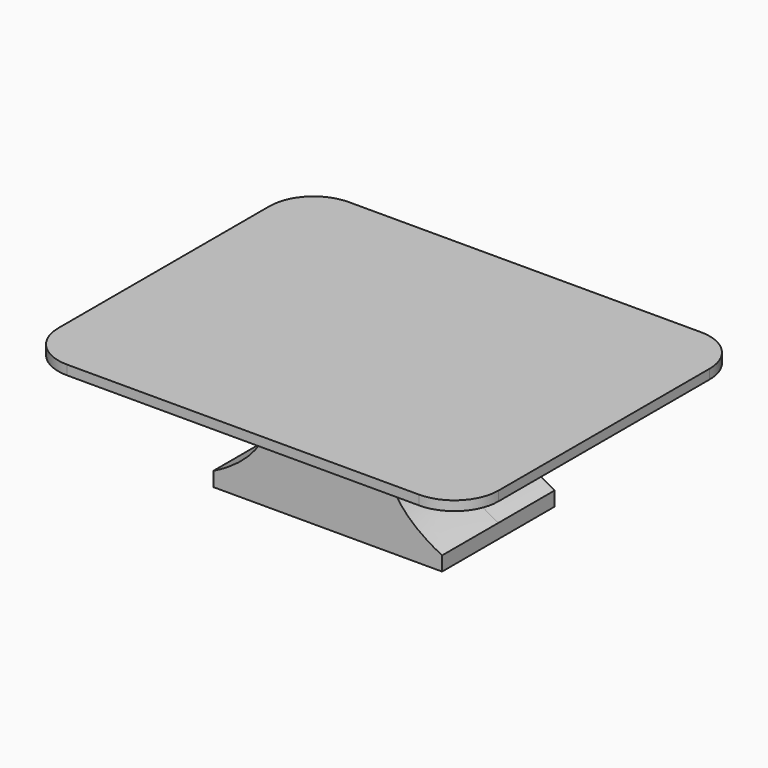
from build123d import *

# Parameters (mm, degrees)
F1_DEPTH     = 20
F2_DEPTH     = 13
F0_W         = 13
F0_H         = 1.6210871795
F3_T4_DEPTH  = 22
F3_T9_DEPTH  = 26
F3_T14_DEPTH = 26
F3_T19_DEPTH = 22
F3_T25_DEPTH = 38.8584149398
F3_T30_DEPTH = 34.8584149398
F3_T38_DEPTH = 34.8584149398
F3_T43_DEPTH = 38.8584149398
F3_T51_DEPTH = 38.8584149398
F3_T56_DEPTH = 34.8584149398
F3_T64_DEPTH = 38.8584149398
F3_T69_DEPTH = 34.8584149398
F4_R         = 5
F5_R         = 5
F7_DEPTH     = 8


# Not quite as in the source:
# - a fillet or chamfer that OpenCascade refuses, or shapes differently, is made with other operations: its cross-section is extruded or revolved along the edge and cut away or added


with BuildPart() as f1:
    # F0 (on Front) → F1 (new body, symmetric)
    with BuildSketch(Plane.XZ):
        Polygon((0, 13.7715177082), (0, 14.85), (-25, 14.85), (-25, 13.7715177082), (-11, 13.7715177082), align=None)
        Polygon((25, 14.85), (0, 14.85), (0, 13.7715177082), (11, 13.7715177082), (25, 13.7715177082), align=None)
    extrude(amount=F1_DEPTH, both=True)

    # F0 (on Front) → F2 (join, symmetric)
    with BuildSketch(Plane.XZ):
        Polygon((0, 12.6210871795), (0, 13.7715177082), (-11, 13.7715177082), (-11, 12.6210871795), (-5.5, 12.6210871795), align=None)
        Polygon((11, 13.7715177082), (0, 13.7715177082), (0, 12.6210871795), (5.5, 12.6210871795), (11, 12.6210871795), align=None)
    extrude(amount=F2_DEPTH, both=True)

    # F3: chamfer of 5 on 4 edges, made by hand


with BuildPart() as f2:
    # F0 (on Front) → F2, piece 2 (new body, symmetric)
    with BuildSketch(Plane.XZ):
        with Locations((-6.5, 0.8105435898)):
            Rectangle(F0_W, F0_H)
        with Locations((6.5, 0.8105435898)):
            Rectangle(F0_W, F0_H)
    extrude(amount=F2_DEPTH, both=True)

    # F4
    f4_edges = [f2.edges().sort_by_distance(p)[0] for p in [
        (-13, 13, 0.810544),
        (-13, -13, 0.810544),
        (13, -13, 0.810544),
        (13, 13, 0.810544),
    ]]
    fillet(f4_edges, radius=F4_R)


with BuildPart() as f3_tool2:
    # F3_s3 → F3_t4 (new body)
    with BuildSketch(Plane.YZ.offset(-11)):
        with BuildLine():
            Line((13.1414213562, 17.7625085358), (7.8585786438, 12.4796658233))
            Line((7.8585786438, 12.4796658233), (7.8585786438, 12.3796658233))
            ThreePointArc((7.8585786438, 12.3796658233), (10.4292893219, 12.5210871795), (13, 12.5210871795))
            Line((13, 12.5210871795), (13.1, 12.6210871795))
            ThreePointArc((13.1, 12.6210871795), (13.1, 15.1917978577), (13.2414213562, 17.7625085358))
            Line((13.2414213562, 17.7625085358), (13.1414213562, 17.7625085358))
        make_face()
    extrude(amount=F3_T4_DEPTH)

    split(bisect_by=Plane.XY.offset(13.7715177082), keep=Keep.BOTTOM)


with BuildPart() as f1_1:
    add(f1.part)

    # F3_t1: cut F3_tool2
    add(f3_tool2.part, mode=Mode.SUBTRACT)


with BuildPart() as f3_tool7:
    # F3_s8 → F3_t9 (new body)
    with BuildSketch(Plane.XZ.offset(-13)):
        with BuildLine():
            Line((-11.1414213562, 17.7625085358), (-5.8585786438, 12.4796658233))
            Line((-5.8585786438, 12.4796658233), (-5.8585786438, 12.3796658233))
            ThreePointArc((-5.8585786438, 12.3796658233), (-8.4292893219, 12.5210871795), (-11, 12.5210871795))
            Line((-11, 12.5210871795), (-11.1, 12.6210871795))
            ThreePointArc((-11.1, 12.6210871795), (-11.1, 15.1917978577), (-11.2414213562, 17.7625085358))
            Line((-11.2414213562, 17.7625085358), (-11.1414213562, 17.7625085358))
        make_face()
    extrude(amount=F3_T9_DEPTH)

    split(bisect_by=Plane.XY.offset(13.7715177082), keep=Keep.BOTTOM)


with BuildPart() as f1_2:
    add(f1_1.part)

    # F3_t6: cut F3_tool7
    add(f3_tool7.part, mode=Mode.SUBTRACT)


with BuildPart() as f3_tool12:
    # F3_s13 → F3_t14 (new body)
    with BuildSketch(Plane.XZ.offset(-13)):
        with BuildLine():
            Line((11.1414213562, 17.7625085358), (5.8585786438, 12.4796658233))
            Line((5.8585786438, 12.4796658233), (5.8585786438, 12.3796658233))
            ThreePointArc((5.8585786438, 12.3796658233), (8.4292893219, 12.5210871795), (11, 12.5210871795))
            Line((11, 12.5210871795), (11.1, 12.6210871795))
            ThreePointArc((11.1, 12.6210871795), (11.1, 15.1917978577), (11.2414213562, 17.7625085358))
            Line((11.2414213562, 17.7625085358), (11.1414213562, 17.7625085358))
        make_face()
    extrude(amount=F3_T14_DEPTH)

    split(bisect_by=Plane.XY.offset(13.7715177082), keep=Keep.BOTTOM)


with BuildPart() as f1_3:
    add(f1_2.part)

    # F3_t11: cut F3_tool12
    add(f3_tool12.part, mode=Mode.SUBTRACT)


with BuildPart() as f3_tool17:
    # F3_s18 → F3_t19 (new body)
    with BuildSketch(Plane.YZ.offset(-11)):
        with BuildLine():
            Line((-13.1414213562, 17.7625085358), (-7.8585786438, 12.4796658233))
            Line((-7.8585786438, 12.4796658233), (-7.8585786438, 12.3796658233))
            ThreePointArc((-7.8585786438, 12.3796658233), (-10.4292893219, 12.5210871795), (-13, 12.5210871795))
            Line((-13, 12.5210871795), (-13.1, 12.6210871795))
            ThreePointArc((-13.1, 12.6210871795), (-13.1, 15.1917978577), (-13.2414213562, 17.7625085358))
            Line((-13.2414213562, 17.7625085358), (-13.1414213562, 17.7625085358))
        make_face()
    extrude(amount=F3_T19_DEPTH)

    split(bisect_by=Plane.XY.offset(13.7715177082), keep=Keep.BOTTOM)


with BuildPart() as f1_4:
    add(f1_3.part)

    # F3_t16: cut F3_tool17
    add(f3_tool17.part, mode=Mode.SUBTRACT)


with BuildPart() as f3_tool23:
    # F3_s24 → F3_t25 (new body)
    with BuildSketch(Plane.XZ.offset(-25.8584149398)):
        with BuildLine():
            Line((-11.1414213562, 17.7625085358), (-5.8585786438, 12.4796658233))
            Line((-5.8585786438, 12.4796658233), (-5.8585786438, 12.3796658233))
            ThreePointArc((-5.8585786438, 12.3796658233), (-8.4292893219, 12.5210871795), (-11, 12.5210871795))
            Line((-11, 12.5210871795), (-11.1, 12.6210871795))
            ThreePointArc((-11.1, 12.6210871795), (-11.1, 15.1917978577), (-11.2414213562, 17.7625085358))
            Line((-11.2414213562, 17.7625085358), (-11.1414213562, 17.7625085358))
        make_face()
    extrude(amount=F3_T25_DEPTH)

    split(bisect_by=Plane.XY.offset(13.7715177082), keep=Keep.BOTTOM)

    split(bisect_by=Plane.XZ.offset(-13), keep=Keep.BOTTOM)


with BuildPart() as f3_tool28:
    # F3_s29 → F3_t30 (new body)
    with BuildSketch(Plane.YZ.offset(-23.8584149398)):
        with BuildLine():
            Line((13.1414213562, 17.7625085358), (7.8585786438, 12.4796658233))
            Line((7.8585786438, 12.4796658233), (7.8585786438, 12.3796658233))
            ThreePointArc((7.8585786438, 12.3796658233), (10.4292893219, 12.5210871795), (13, 12.5210871795))
            Line((13, 12.5210871795), (13.1, 12.6210871795))
            ThreePointArc((13.1, 12.6210871795), (13.1, 15.1917978577), (13.2414213562, 17.7625085358))
            Line((13.2414213562, 17.7625085358), (13.1414213562, 17.7625085358))
        make_face()
    extrude(amount=F3_T30_DEPTH)

    split(bisect_by=Plane.XY.offset(13.7715177082), keep=Keep.BOTTOM)

    split(bisect_by=Plane.YZ.offset(-11), keep=Keep.BOTTOM)


with BuildPart() as f3_tool23_1:
    add(f3_tool23.part)

    # F3_t33: intersect F3_tool28
    add(f3_tool28.part, mode=Mode.INTERSECT)


with BuildPart() as f1_5:
    add(f1_4.part)

    # F3_t21: cut F3_tool23
    add(f3_tool23_1.part, mode=Mode.SUBTRACT)


with BuildPart() as f3_tool36:
    # F3_s37 → F3_t38 (new body)
    with BuildSketch(Plane.YZ.offset(-11)):
        with BuildLine():
            Line((13.1414213562, 17.7625085358), (7.8585786438, 12.4796658233))
            Line((7.8585786438, 12.4796658233), (7.8585786438, 12.3796658233))
            ThreePointArc((7.8585786438, 12.3796658233), (10.4292893219, 12.5210871795), (13, 12.5210871795))
            Line((13, 12.5210871795), (13.1, 12.6210871795))
            ThreePointArc((13.1, 12.6210871795), (13.1, 15.1917978577), (13.2414213562, 17.7625085358))
            Line((13.2414213562, 17.7625085358), (13.1414213562, 17.7625085358))
        make_face()
    extrude(amount=F3_T38_DEPTH)

    split(bisect_by=Plane.XY.offset(13.7715177082), keep=Keep.BOTTOM)

    split(bisect_by=Plane.YZ.offset(11), keep=Keep.TOP)


with BuildPart() as f3_tool41:
    # F3_s42 → F3_t43 (new body)
    with BuildSketch(Plane.XZ.offset(-25.8584149398)):
        with BuildLine():
            Line((11.1414213562, 17.7625085358), (5.8585786438, 12.4796658233))
            Line((5.8585786438, 12.4796658233), (5.8585786438, 12.3796658233))
            ThreePointArc((5.8585786438, 12.3796658233), (8.4292893219, 12.5210871795), (11, 12.5210871795))
            Line((11, 12.5210871795), (11.1, 12.6210871795))
            ThreePointArc((11.1, 12.6210871795), (11.1, 15.1917978577), (11.2414213562, 17.7625085358))
            Line((11.2414213562, 17.7625085358), (11.1414213562, 17.7625085358))
        make_face()
    extrude(amount=F3_T43_DEPTH)

    split(bisect_by=Plane.XY.offset(13.7715177082), keep=Keep.BOTTOM)

    split(bisect_by=Plane.XZ.offset(-13), keep=Keep.BOTTOM)


with BuildPart() as f3_tool36_1:
    add(f3_tool36.part)

    # F3_t46: intersect F3_tool41
    add(f3_tool41.part, mode=Mode.INTERSECT)


with BuildPart() as f1_6:
    add(f1_5.part)

    # F3_t34: cut F3_tool36
    add(f3_tool36_1.part, mode=Mode.SUBTRACT)


with BuildPart() as f3_tool49:
    # F3_s50 → F3_t51 (new body)
    with BuildSketch(Plane.XZ.offset(-13)):
        with BuildLine():
            Line((-11.1414213562, 17.7625085358), (-5.8585786438, 12.4796658233))
            Line((-5.8585786438, 12.4796658233), (-5.8585786438, 12.3796658233))
            ThreePointArc((-5.8585786438, 12.3796658233), (-8.4292893219, 12.5210871795), (-11, 12.5210871795))
            Line((-11, 12.5210871795), (-11.1, 12.6210871795))
            ThreePointArc((-11.1, 12.6210871795), (-11.1, 15.1917978577), (-11.2414213562, 17.7625085358))
            Line((-11.2414213562, 17.7625085358), (-11.1414213562, 17.7625085358))
        make_face()
    extrude(amount=F3_T51_DEPTH)

    split(bisect_by=Plane.XY.offset(13.7715177082), keep=Keep.BOTTOM)

    split(bisect_by=Plane.XZ.offset(13), keep=Keep.TOP)


with BuildPart() as f3_tool54:
    # F3_s55 → F3_t56 (new body)
    with BuildSketch(Plane.YZ.offset(-23.8584149398)):
        with BuildLine():
            Line((-13.1414213562, 17.7625085358), (-7.8585786438, 12.4796658233))
            Line((-7.8585786438, 12.4796658233), (-7.8585786438, 12.3796658233))
            ThreePointArc((-7.8585786438, 12.3796658233), (-10.4292893219, 12.5210871795), (-13, 12.5210871795))
            Line((-13, 12.5210871795), (-13.1, 12.6210871795))
            ThreePointArc((-13.1, 12.6210871795), (-13.1, 15.1917978577), (-13.2414213562, 17.7625085358))
            Line((-13.2414213562, 17.7625085358), (-13.1414213562, 17.7625085358))
        make_face()
    extrude(amount=F3_T56_DEPTH)

    split(bisect_by=Plane.XY.offset(13.7715177082), keep=Keep.BOTTOM)

    split(bisect_by=Plane.YZ.offset(-11), keep=Keep.BOTTOM)


with BuildPart() as f3_tool49_1:
    add(f3_tool49.part)

    # F3_t59: intersect F3_tool54
    add(f3_tool54.part, mode=Mode.INTERSECT)


with BuildPart() as f1_7:
    add(f1_6.part)

    # F3_t47: cut F3_tool49
    add(f3_tool49_1.part, mode=Mode.SUBTRACT)


with BuildPart() as f3_tool62:
    # F3_s63 → F3_t64 (new body)
    with BuildSketch(Plane.XZ.offset(-13)):
        with BuildLine():
            Line((11.1414213562, 17.7625085358), (5.8585786438, 12.4796658233))
            Line((5.8585786438, 12.4796658233), (5.8585786438, 12.3796658233))
            ThreePointArc((5.8585786438, 12.3796658233), (8.4292893219, 12.5210871795), (11, 12.5210871795))
            Line((11, 12.5210871795), (11.1, 12.6210871795))
            ThreePointArc((11.1, 12.6210871795), (11.1, 15.1917978577), (11.2414213562, 17.7625085358))
            Line((11.2414213562, 17.7625085358), (11.1414213562, 17.7625085358))
        make_face()
    extrude(amount=F3_T64_DEPTH)

    split(bisect_by=Plane.XY.offset(13.7715177082), keep=Keep.BOTTOM)

    split(bisect_by=Plane.XZ.offset(13), keep=Keep.TOP)


with BuildPart() as f3_tool67:
    # F3_s68 → F3_t69 (new body)
    with BuildSketch(Plane.YZ.offset(-11)):
        with BuildLine():
            Line((-13.1414213562, 17.7625085358), (-7.8585786438, 12.4796658233))
            Line((-7.8585786438, 12.4796658233), (-7.8585786438, 12.3796658233))
            ThreePointArc((-7.8585786438, 12.3796658233), (-10.4292893219, 12.5210871795), (-13, 12.5210871795))
            Line((-13, 12.5210871795), (-13.1, 12.6210871795))
            ThreePointArc((-13.1, 12.6210871795), (-13.1, 15.1917978577), (-13.2414213562, 17.7625085358))
            Line((-13.2414213562, 17.7625085358), (-13.1414213562, 17.7625085358))
        make_face()
    extrude(amount=F3_T69_DEPTH)

    split(bisect_by=Plane.XY.offset(13.7715177082), keep=Keep.BOTTOM)

    split(bisect_by=Plane.YZ.offset(11), keep=Keep.TOP)


with BuildPart() as f3_tool62_1:
    add(f3_tool62.part)

    # F3_t72: intersect F3_tool67
    add(f3_tool67.part, mode=Mode.INTERSECT)


with BuildPart() as f1_8:
    add(f1_7.part)

    # F3_t60: cut F3_tool62
    add(f3_tool62_1.part, mode=Mode.SUBTRACT)

    # F5
    f5_edges = [f1_8.edges().sort_by_distance(p)[0] for p in [
        (-25, -20, 14.310759),
        (-25, 20, 14.310759),
        (25, -20, 14.310759),
        (25, 20, 14.310759),
    ]]
    fillet(f5_edges, radius=F5_R)

    # F0 (on Front) → F7 (join, symmetric)
    with BuildSketch(Plane.XZ):
        with BuildLine():
            Line((0, 1.6210871795), (0, 12.6210871795))
            Line((0, 12.6210871795), (-5.5, 12.6210871795))
            add(Edge.make_bspline(
                [(-13, 1.6210871795), (-9.1716769267, 3.5339947176), (-6.259098086, 6.2224261798), (-5.5, 12.6210871795)],
                knots=[0, 0, 0, 0, 13.3135269557, 13.3135269557, 13.3135269557, 13.3135269557], degree=3))
            Line((-13, 1.6210871795), (0, 1.6210871795))
        make_face()
        with Locations((-6.5, 0.8105435898)):
            Rectangle(F0_W, F0_H)
        with BuildLine():
            Line((5.5, 12.6210871795), (0, 12.6210871795))
            Line((0, 12.6210871795), (0, 1.6210871795))
            Line((0, 1.6210871795), (13, 1.6210871795))
            add(Edge.make_bspline(
                [(13, 1.6210871795), (9.1716769267, 3.5339947176), (6.259098086, 6.2224261798), (5.5, 12.6210871795)],
                knots=[0, 0, 0, 0, 13.3135269557, 13.3135269557, 13.3135269557, 13.3135269557], degree=3))
        make_face()
        with Locations((6.5, 0.8105435898)):
            Rectangle(F0_W, F0_H)
    extrude(amount=F7_DEPTH, both=True)


solid = f1_8.part
